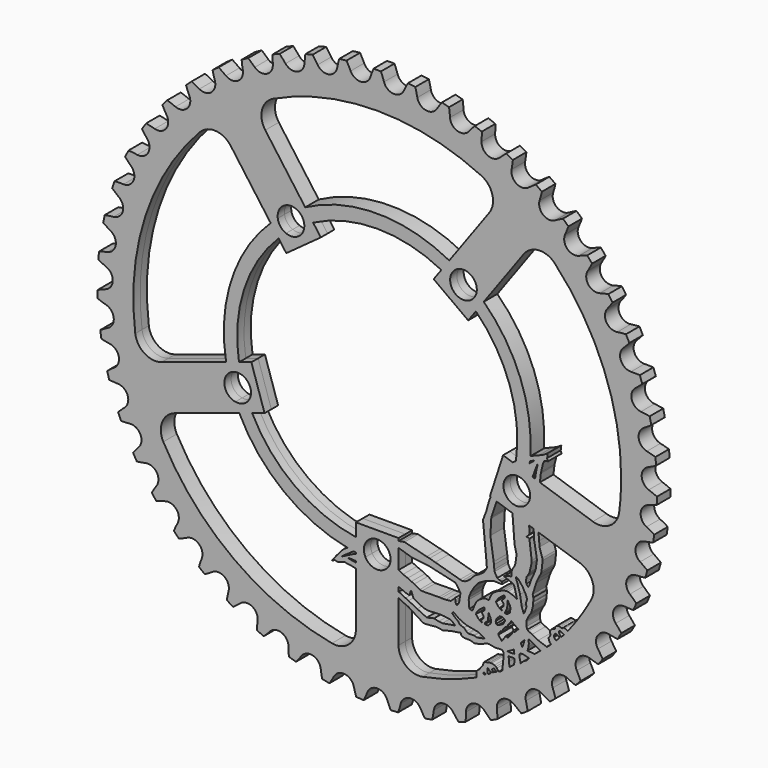
from build123d import *

# Parameters (mm, degrees)
F0_R     = 95.23914061
F2_DEPTH = 3.175
F3_DEPTH = 3.175


# Not quite as in the source:
# - a length typed as a fraction of an inch, garbled in the dataset ("3 / 203.2 mm" for 3/8 in), is restored


with BuildPart() as f2:
    # F0 (on Front) → F2 (new body, symmetric)
    with BuildSketch(Plane.XZ):
        with BuildLine():
            ThreePointArc((1.3974512393, 104.8471286678), (0, 104.8564411939), (-1.3974512393, 104.8471286678))
            ThreePointArc((-1.3974512393, 104.8471286678), (-1.9989055088, 103.3019703404), (-2.5462079028, 101.7368116953))
            ThreePointArc((-2.5462079028, 101.7368116953), (-3.9052398194, 99.8191421504), (-6.1056801538, 98.9930146972))
            ThreePointArc((-6.1056801538, 98.9930146972), (-8.3909636625, 99.5424721739), (-9.9753539423, 101.2785976519))
            ThreePointArc((-9.9753539423, 101.2785976519), (-10.7108477336, 102.7646361365), (-11.4976251519, 104.2241712642))
            ThreePointArc((-11.4976251519, 104.2241712642), (-12.8856288235, 104.061682812), (-14.2713436942, 103.880710476))
            ThreePointArc((-14.2713436942, 103.880710476), (-14.6783573813, 102.2733519742), (-15.0291718315, 100.6527993782))
            ThreePointArc((-15.0291718315, 100.6527993782), (-16.1422438465, 98.5826556819), (-18.224484574, 97.4923815023))
            ThreePointArc((-18.224484574, 97.4923815023), (-20.5599686886, 97.7568397874), (-22.34569959, 99.2851033058))
            ThreePointArc((-22.34569959, 99.2851033058), (-23.2582354424, 100.6694948013), (-24.2184092659, 102.0212816645))
            ThreePointArc((-24.2184092659, 102.0212816645), (-25.5759246489, 101.6894553933), (-26.9288971262, 101.3395666036))
            ThreePointArc((-26.9288971262, 101.3395666036), (-27.1353003181, 99.6943738437), (-27.2843088352, 98.0429932223))
            ThreePointArc((-27.2843088352, 98.0429932223), (-28.1345479113, 95.8517566428), (-30.0670243851, 94.5138631821))
            ThreePointArc((-30.0670243851, 94.5138631821), (-32.417305547, 94.4893133574), (-34.3773072098, 95.7865479992))
            ThreePointArc((-34.3773072098, 95.7865479992), (-35.45305201, 97.0483065417), (-36.5720669823, 98.2718534296))
            ThreePointArc((-36.5720669823, 98.2718534296), (-37.8785155273, 97.7757194874), (-39.1782359275, 97.2622182014))
            ThreePointArc((-39.1782359275, 97.2622182014), (-39.1808997623, 95.6041306286), (-39.125843529, 93.9469552287))
            ThreePointArc((-39.125843529, 93.9469552287), (-39.7003609085, 91.667842679), (-41.4537787551, 90.1026110382))
            ThreePointArc((-41.4537787551, 90.1026110382), (-43.7832290977, 89.7894252541), (-45.8877898946, 90.8359662645))
            ThreePointArc((-45.8877898946, 90.8359662645), (-47.110436448, 91.9559648806), (-48.3713294427, 93.0327240695))
            ThreePointArc((-48.3713294427, 93.0327240695), (-49.6069067216, 92.3798033412), (-50.8336726082, 91.7104737148))
            ThreePointArc((-50.8336726082, 91.7104737148), (-50.632556705, 90.0646262467), (-50.3742703176, 88.4267771581))
            ThreePointArc((-50.3742703176, 88.4267771581), (-50.6643569028, 86.0943376612), (-52.2121360949, 84.3254951565))
            ThreePointArc((-52.2121360949, 84.3254951565), (-54.4854435255, 83.7284209902), (-56.70266046, 84.5084038742))
            ThreePointArc((-56.70266046, 84.5084038742), (-58.0536746912, 85.4696645266), (-59.4373318558, 86.3833134448))
            ThreePointArc((-59.4373318558, 86.3833134448), (-60.5833077764, 85.5835035431), (-61.7185226292, 84.7684919313))
            ThreePointArc((-61.7185226292, 84.7684919313), (-61.3166757, 83.1598339377), (-60.8590745169, 81.5661392831))
            ThreePointArc((-60.8590745169, 81.5661392831), (-60.8603328907, 79.2157302442), (-62.1790106736, 77.2700907249))
            ThreePointArc((-62.1790106736, 77.2700907249), (-64.3617141688, 76.3981792122), (-66.6579764924, 76.8997802243))
            ThreePointArc((-66.6579764924, 76.8997802243), (-68.1168784028, 77.6877311814), (-69.6023249051, 78.4244198426))
            ThreePointArc((-69.6023249051, 78.4244198426), (-70.6413276406, 77.4898450703), (-71.6677827595, 76.5415062183))
            ThreePointArc((-71.6677827595, 76.5415062183), (-71.0712963941, 74.9944233147), (-70.4213171828, 73.4690418805))
            ThreePointArc((-70.4213171828, 73.4690418805), (-70.1337282697, 71.1362931047), (-71.2033148323, 69.0433504827))
            ThreePointArc((-71.2033148323, 69.0433504827), (-73.2623268321, 67.9098189133), (-75.6028255485, 68.1254342936))
            ThreePointArc((-75.6028255485, 68.1254342936), (-77.1474996722, 68.7281310219), (-78.7122176575, 69.276691977))
            ThreePointArc((-78.7122176575, 69.276691977), (-79.6284969855, 68.221519535), (-80.5306323574, 67.1542292932))
            ThreePointArc((-80.5306323574, 67.1542292932), (-79.748548681, 65.6921736793), (-78.9160444638, 64.2582286932))
            ThreePointArc((-78.9160444638, 64.2582286932), (-78.3439678185, 61.9785022741), (-79.1482493188, 59.7699834261))
            ThreePointArc((-79.1482493188, 59.7699834261), (-81.0523573, 58.3920149832), (-83.4016128346, 58.3183762222))
            ThreePointArc((-83.4016128346, 58.3183762222), (-85.0086434865, 58.7266824538), (-86.628913425, 59.0788000779))
            ThreePointArc((-86.628913425, 59.0788000779), (-87.408579485, 57.9190253048), (-88.172719657, 56.7489627052))
            ThreePointArc((-88.172719657, 56.7489627052), (-87.2168942611, 55.3940976539), (-86.2144849533, 54.0733262601))
            ThreePointArc((-86.2144849533, 54.0733262601), (-85.3665926745, 51.8811805265), (-85.8933770249, 49.5905643469))
            ThreePointArc((-85.8933770249, 49.5905643469), (-87.6137166516, 47.9890476274), (-89.9361166851, 47.6272710137))
            ThreePointArc((-89.9361166851, 47.6272710137), (-91.5811429185, 47.8349972424), (-93.2324031697, 47.9853337911))
            ThreePointArc((-93.2324031697, 47.9853337911), (-93.8636370189, 46.7385376903), (-94.478198405, 45.4834396894))
            ThreePointArc((-94.478198405, 45.4834396894), (-93.3631206282, 44.2563035737), (-92.2060017332, 43.0687273203))
            ThreePointArc((-92.2060017332, 43.0687273203), (-91.0951470036, 40.9973929669), (-91.3364486902, 38.6594028621))
            ThreePointArc((-91.3364486902, 38.6594028621), (-92.8469413671, 36.858615227), (-95.1072806824, 36.2141849253))
            ThreePointArc((-95.1072806824, 36.2141849253), (-96.7653655766, 36.2181822331), (-98.4225847182, 36.1644587577))
            ThreePointArc((-98.4225847182, 36.1644587577), (-98.8958174949, 34.8495414871), (-99.351483971, 33.5284340911))
            ThreePointArc((-99.351483971, 33.5284340911), (-98.0940572557, 32.4476290436), (-96.7997695163, 31.4112503761))
            ThreePointArc((-96.7997695163, 31.4112503761), (-95.4427917614, 29.4921267203), (-95.3949528966, 27.1422042371))
            ThreePointArc((-95.3949528966, 27.1422042371), (-96.6727010946, 25.1694437913), (-98.8367152516, 24.252128708))
            ThreePointArc((-98.8367152516, 24.252128708), (-100.4827239298, 24.0523364999), (-102.1207802088, 23.7953673935))
            ThreePointArc((-102.1207802088, 23.7953673935), (-102.4288381865, 22.4322617587), (-102.7187023133, 21.065171609))
            ThreePointArc((-102.7187023133, 21.065171609), (-101.3379879668, 20.1470815326), (-99.9261514659, 19.2776108951))
            ThreePointArc((-99.9261514659, 19.2776108951), (-98.343621085, 17.5397898952), (-98.0073668573, 15.2135574631))
            ThreePointArc((-98.0073668573, 15.2135574631), (-99.0330012161, 13.0987292441), (-101.0678859662, 11.9224349409))
            ThreePointArc((-101.0678859662, 11.9224349409), (-102.6768666145, 11.5218818629), (-104.2709287676, 11.0655625153))
            ThreePointArc((-104.2709287676, 11.0655625153), (-104.4091421014, 9.6749318081), (-104.5288098342, 8.2825825979))
            ThreePointArc((-104.5288098342, 8.2825825979), (-103.0457380786, 7.5411248023), (-101.5377548183, 6.8517424834))
            ThreePointArc((-101.5377548183, 6.8517424834), (-99.753661359, 5.3215677344), (-99.1340890397, 3.0542886658))
            ThreePointArc((-99.1340890397, 3.0542886658), (-99.8920619879, 0.8294513136), (-101.7669705525, -0.5879907869))
            ThreePointArc((-101.7669705525, -0.5879907869), (-103.3145326645, -1.1832327583), (-104.8404363343, -1.831985011))
            ThreePointArc((-104.8404363343, -1.831985011), (-104.8067098509, -3.2290602466), (-104.7543671488, -4.6255619225))
            ThreePointArc((-104.7543671488, -4.6255619225), (-103.1914198401, -5.1791476929), (-101.6101493096, -5.67799136))
            ThreePointArc((-101.6101493096, -5.67799136), (-99.6515378101, -6.9773239687), (-98.758039484, -9.1512800343))
            ThreePointArc((-98.758039484, -9.1512800343), (-99.2368609244, -11.4524002533), (-100.9233716008, -13.0895031738))
            ThreePointArc((-100.9233716008, -13.0895031738), (-102.3860557123, -13.870410777), (-103.8206697546, -14.701761512))
            ThreePointArc((-103.8206697546, -14.701761512), (-103.6155147131, -16.0841030394), (-103.3919550381, -17.4635876392))
            ThreePointArc((-103.3919550381, -17.4635876392), (-101.7728248644, -17.8209095885), (-100.142237513, -18.1216526423))
            ThreePointArc((-100.142237513, -18.1216526423), (-98.0387985272, -19.1704465528), (-96.8849187181, -21.2181246574))
            ThreePointArc((-96.8849187181, -21.2181246574), (-97.0773302057, -23.5606451062), (-98.5498772112, -25.3925920352))
            ThreePointArc((-98.5498772112, -25.3925920352), (-99.9055105221, -26.3473275071), (-101.2270876503, -27.3486742946))
            ThreePointArc((-101.2270876503, -27.3486742946), (-100.8536139921, -28.6953272254), (-100.4622262811, -30.0368831687))
            ThreePointArc((-100.4622262811, -30.0368831687), (-98.8114576053, -30.1925246603), (-97.1562714752, -30.2906081427))
            ThreePointArc((-97.1562714752, -30.2906081427), (-94.9398909938, -31.0729647084), (-93.5431213435, -32.9633241392))
            ThreePointArc((-93.5431213435, -32.9633241392), (-93.4462061162, -35.3117345958), (-94.6824671393, -37.3107550852))
            ThreePointArc((-94.6824671393, -37.3107550852), (-95.9104996304, -38.4248456091), (-97.0990060825, -39.5810090527))
            ThreePointArc((-97.0990060825, -39.5810090527), (-96.5628752875, -40.8715595011), (-96.0095925791, -42.1548501673))
            ThreePointArc((-96.0095925791, -42.1548501673), (-94.3522093717, -42.1064518349), (-92.6975153974, -42.0003889001))
            ThreePointArc((-92.6975153974, -42.0003889001), (-90.4017914894, -42.504448393), (-88.7833056019, -44.2088332281))
            ThreePointArc((-88.7833056019, -44.2088332281), (-88.3985327959, -46.5275341837), (-89.3797673795, -48.6633251205))
            ThreePointArc((-89.3797673795, -48.6633251205), (-90.4615833302, -49.9198822198), (-91.4990025598, -51.2133360601))
            ThreePointArc((-91.4990025598, -51.2133360601), (-90.8083418243, -52.4282205969), (-90.1015513205, -53.6337926077))
            ThreePointArc((-90.1015513205, -53.6337926077), (-88.4626778214, -53.3820881206), (-86.8335594768, -53.0734865747))
            ThreePointArc((-86.8335594768, -53.0734865747), (-84.4932929765, -53.2916079667), (-82.6776254481, -54.7841814692))
            ThreePointArc((-82.6776254481, -54.7841814692), (-82.0108278269, -57.0380237809), (-82.722161455, -59.2782087517))
            ThreePointArc((-82.722161455, -59.2782087517), (-83.6413616381, -60.6581843016), (-84.5119674272, -62.0693210969))
            ThreePointArc((-84.5119674272, -62.0693210969), (-83.677246464, -63.1901233109), (-82.8276623883, -64.2997014234))
            ThreePointArc((-82.8276623883, -64.2997014234), (-81.2321422492, -63.8485063651), (-79.6532953078, -63.342044293))
            ThreePointArc((-79.6532953078, -63.342044293), (-77.3039622698, -63.270921086), (-75.3186367695, -64.5290573631))
            ThreePointArc((-75.3186367695, -64.5290573631), (-74.3799223052, -66.683875079), (-74.8105718852, -68.9944951631))
            ThreePointArc((-74.8105718852, -68.9944951631), (-75.5532221629, -70.476970141), (-76.2438170152, -71.9843984958))
            ThreePointArc((-76.2438170152, -71.9843984958), (-75.2776893432, -72.9941281679), (-74.2981905242, -73.990892309))
            ThreePointArc((-74.2981905242, -73.990892309), (-72.770210204, -73.3470463367), (-71.265568376, -72.6504011871))
            ThreePointArc((-71.265568376, -72.6504011871), (-68.9427822944, -72.2911115366), (-66.817894333, -73.2957385248))
            ThreePointArc((-66.817894333, -73.2957385248), (-65.6214929802, -75.3188668047), (-65.7649303033, -77.664895357))
            ThreePointArc((-65.7649303033, -77.664895357), (-66.3197728544, -79.2273969532), (-66.8198880558, -80.8082657904))
            ThreePointArc((-66.8198880558, -80.8082657904), (-65.7369991858, -81.691616448), (-64.6424338271, -82.5604566893))
            ThreePointArc((-64.6424338271, -82.5604566893), (-63.20515595, -81.7337198516), (-61.7975280718, -80.857452055))
            ThreePointArc((-61.7975280718, -80.857452055), (-59.5365000158, -80.2154424257), (-57.3042607288, -80.9513310039))
            ThreePointArc((-57.3042607288, -80.9513310039), (-55.8683087124, -82.8121012854), (-55.7223594151, -85.1579749044))
            ThreePointArc((-55.7223594151, -85.1579749044), (-56.0809833921, -86.7768171877), (-56.3830377061, -88.407162147))
            ThreePointArc((-56.3830377061, -88.407162147), (-55.1998031293, -89.1507430946), (-54.006763726, -89.8784887038))
            ThreePointArc((-54.006763726, -89.8784887038), (-52.6819759595, -88.8813934884), (-51.3927002349, -87.8387863712))
            ThreePointArc((-51.3927002349, -87.8387863712), (-49.2277050852, -86.9237889748), (-46.9219529448, -87.3797838223))
            ThreePointArc((-46.9219529448, -87.3797838223), (-45.2682178335, -89.0499887246), (-44.8350943583, -91.3601463576))
            ThreePointArc((-44.8350943583, -91.3601463576), (-44.9920633874, -93.0107893289), (-45.0914779783, -94.6658960427))
            ThreePointArc((-45.0914779783, -94.6658960427), (-43.825834325, -95.2584353512), (-42.5524061384, -95.8340544466))
            ThreePointArc((-42.5524061384, -95.8340544466), (-41.3601909146, -94.6817158006), (-40.2088114494, -93.488574224))
            ThreePointArc((-40.2088114494, -93.488574224), (-38.1726683254, -92.3144594882), (-35.8283561837, -92.483648188))
            ThreePointArc((-35.8283561837, -92.483648188), (-33.9819069162, -93.9379691074), (-33.2681749735, -96.1773911194))
            ThreePointArc((-33.2681749735, -96.1773911194), (-33.2211095641, -97.834812714), (-33.1163774082, -99.4895914516))
            ThreePointArc((-33.1163774082, -99.4895914516), (-31.7875105459, -99.9221068289), (-30.4529974492, -100.3368736118))
            ThreePointArc((-30.4529974492, -100.3368736118), (-29.4114275356, -99.0467598146), (-28.4153980688, -97.7211705886))
            ThreePointArc((-28.4153980688, -97.7211705886), (-26.5389728249, -96.305736896), (-24.1916380643, -96.1855547198))
            ThreePointArc((-24.1916380643, -96.1855547198), (-22.1804649293, -97.4019456336), (-21.1969439678, -99.5366846697))
            ThreePointArc((-21.1969439678, -99.5366846697), (-20.9465575835, -101.1757600656), (-20.6392663135, -102.8051260681))
            ThreePointArc((-20.6392663135, -102.8051260681), (-19.2673205093, -103.0710610221), (-17.8919523608, -103.3186880509))
            ThreePointArc((-17.8919523608, -103.3186880509), (-17.0168168956, -101.9103559124), (-16.1912362186, -100.4724136185))
            ThreePointArc((-16.1912362186, -100.4724136185), (-14.5029735487, -98.8371175011), (-12.1881993714, -98.4293862882))
            ThreePointArc((-12.1881993714, -98.4293862882), (-10.0427897036, -99.38940795), (-8.8043888985, -101.3871035425))
            ThreePointArc((-8.8043888985, -101.3871035425), (-8.3544771417, -102.9829860275), (-7.84928498, -104.5622397672))
            ThreePointArc((-7.84928498, -104.5622397672), (-6.4550575339, -104.6575629951), (-5.0596835126, -104.7342964964))
            ThreePointArc((-5.0596835126, -104.7342964964), (-4.3642486574, -103.2290948963), (-3.7216317317, -101.7005972739))
            ThreePointArc((-3.7216317317, -101.7005972739), (-2.247123977, -99.8702281539), (0, -99.1811286939))
            ThreePointArc((0, -99.1811286939), (2.247123977, -99.8702281539), (3.7216317317, -101.7005972739))
            ThreePointArc((3.7216317317, -101.7005972739), (4.3642486574, -103.2290948963), (5.0596835126, -104.7342964964))
            ThreePointArc((5.0596835126, -104.7342964964), (6.4550575339, -104.6575629951), (7.84928498, -104.5622397672))
            ThreePointArc((7.84928498, -104.5622397672), (8.3544771417, -102.9829860275), (8.8043888985, -101.3871035425))
            ThreePointArc((8.8043888985, -101.3871035425), (10.0427897036, -99.38940795), (12.1881993714, -98.4293862882))
            ThreePointArc((12.1881993714, -98.4293862882), (14.5029735487, -98.8371175011), (16.1912362186, -100.4724136185))
            ThreePointArc((16.1912362186, -100.4724136185), (17.0168168956, -101.9103559124), (17.8919523608, -103.3186880509))
            ThreePointArc((17.8919523608, -103.3186880509), (19.2673205093, -103.0710610221), (20.6392663135, -102.8051260681))
            ThreePointArc((20.6392663135, -102.8051260681), (20.9465575835, -101.1757600656), (21.1969439678, -99.5366846697))
            ThreePointArc((21.1969439678, -99.5366846697), (22.1804649293, -97.4019456336), (24.1916380643, -96.1855547198))
            ThreePointArc((24.1916380643, -96.1855547198), (26.5389728249, -96.305736896), (28.4153980688, -97.7211705886))
            ThreePointArc((28.4153980688, -97.7211705886), (29.4114275356, -99.0467598146), (30.4529974492, -100.3368736118))
            ThreePointArc((30.4529974492, -100.3368736118), (31.7875105459, -99.9221068289), (33.1163774082, -99.4895914516))
            ThreePointArc((33.1163774082, -99.4895914516), (33.2211095641, -97.834812714), (33.2681749735, -96.1773911194))
            ThreePointArc((33.2681749735, -96.1773911194), (33.9819069162, -93.9379691074), (35.8283561837, -92.483648188))
            ThreePointArc((35.8283561837, -92.483648188), (38.1726683254, -92.3144594882), (40.2088114494, -93.488574224))
            ThreePointArc((40.2088114494, -93.488574224), (41.3601909146, -94.6817158006), (42.5524061384, -95.8340544466))
            ThreePointArc((42.5524061384, -95.8340544466), (43.825834325, -95.2584353512), (45.0914779783, -94.6658960427))
            ThreePointArc((45.0914779783, -94.6658960427), (44.9920633874, -93.0107893289), (44.8350943583, -91.3601463576))
            ThreePointArc((44.8350943583, -91.3601463576), (45.2682178335, -89.0499887246), (46.9219529448, -87.3797838223))
            ThreePointArc((46.9219529448, -87.3797838223), (49.2277050852, -86.9237889748), (51.3927002349, -87.8387863712))
            ThreePointArc((51.3927002349, -87.8387863712), (52.6819759595, -88.8813934884), (54.006763726, -89.8784887038))
            ThreePointArc((54.006763726, -89.8784887038), (55.1998031293, -89.1507430946), (56.3830377061, -88.407162147))
            ThreePointArc((56.3830377061, -88.407162147), (56.0809833921, -86.7768171877), (55.7223594151, -85.1579749044))
            ThreePointArc((55.7223594151, -85.1579749044), (55.8683087124, -82.8121012854), (57.3042607288, -80.9513310039))
            ThreePointArc((57.3042607288, -80.9513310039), (59.5365000158, -80.2154424257), (61.7975280718, -80.857452055))
            ThreePointArc((61.7975280718, -80.857452055), (63.20515595, -81.7337198516), (64.6424338271, -82.5604566893))
            ThreePointArc((64.6424338271, -82.5604566893), (65.7369991858, -81.691616448), (66.8198880558, -80.8082657904))
            ThreePointArc((66.8198880558, -80.8082657904), (66.3197728544, -79.2273969532), (65.7649303033, -77.664895357))
            ThreePointArc((65.7649303033, -77.664895357), (65.6214929802, -75.3188668047), (66.817894333, -73.2957385248))
            ThreePointArc((66.817894333, -73.2957385248), (68.9427822944, -72.2911115366), (71.265568376, -72.6504011871))
            ThreePointArc((71.265568376, -72.6504011871), (72.770210204, -73.3470463367), (74.2981905242, -73.990892309))
            ThreePointArc((74.2981905242, -73.990892309), (75.2776893432, -72.9941281679), (76.2438170152, -71.9843984958))
            ThreePointArc((76.2438170152, -71.9843984958), (75.5532221629, -70.476970141), (74.8105718852, -68.9944951631))
            ThreePointArc((74.8105718852, -68.9944951631), (74.3799223052, -66.683875079), (75.3186367695, -64.5290573631))
            ThreePointArc((75.3186367695, -64.5290573631), (77.3039622698, -63.270921086), (79.6532953078, -63.342044293))
            ThreePointArc((79.6532953078, -63.342044293), (81.2321422492, -63.8485063651), (82.8276623883, -64.2997014234))
            ThreePointArc((82.8276623883, -64.2997014234), (83.677246464, -63.1901233109), (84.5119674272, -62.0693210969))
            ThreePointArc((84.5119674272, -62.0693210969), (83.6413616381, -60.6581843016), (82.722161455, -59.2782087517))
            ThreePointArc((82.722161455, -59.2782087517), (82.0108278269, -57.0380237809), (82.6776254481, -54.7841814692))
            ThreePointArc((82.6776254481, -54.7841814692), (84.4932929765, -53.2916079667), (86.8335594768, -53.0734865747))
            ThreePointArc((86.8335594768, -53.0734865747), (88.4626778214, -53.3820881206), (90.1015513205, -53.6337926077))
            ThreePointArc((90.1015513205, -53.6337926077), (90.8083418243, -52.4282205969), (91.4990025598, -51.2133360601))
            ThreePointArc((91.4990025598, -51.2133360601), (90.4615833302, -49.9198822198), (89.3797673795, -48.6633251205))
            ThreePointArc((89.3797673795, -48.6633251205), (88.3985327959, -46.5275341837), (88.7833056019, -44.2088332281))
            ThreePointArc((88.7833056019, -44.2088332281), (90.4017914894, -42.504448393), (92.6975153974, -42.0003889001))
            ThreePointArc((92.6975153974, -42.0003889001), (94.3522093717, -42.1064518349), (96.0095925791, -42.1548501673))
            ThreePointArc((96.0095925791, -42.1548501673), (96.5628752875, -40.8715595011), (97.0990060825, -39.5810090527))
            ThreePointArc((97.0990060825, -39.5810090527), (95.9104996304, -38.4248456091), (94.6824671393, -37.3107550852))
            ThreePointArc((94.6824671393, -37.3107550852), (93.4462061162, -35.3117345958), (93.5431213435, -32.9633241392))
            ThreePointArc((93.5431213435, -32.9633241392), (94.9398909938, -31.0729647084), (97.1562714752, -30.2906081427))
            ThreePointArc((97.1562714752, -30.2906081427), (98.8114576053, -30.1925246603), (100.4622262811, -30.0368831687))
            ThreePointArc((100.4622262811, -30.0368831687), (100.8536139921, -28.6953272254), (101.2270876503, -27.3486742946))
            ThreePointArc((101.2270876503, -27.3486742946), (99.9055105221, -26.3473275071), (98.5498772112, -25.3925920352))
            ThreePointArc((98.5498772112, -25.3925920352), (97.0773302057, -23.5606451062), (96.8849187181, -21.2181246574))
            ThreePointArc((96.8849187181, -21.2181246574), (98.0387985272, -19.1704465528), (100.142237513, -18.1216526423))
            ThreePointArc((100.142237513, -18.1216526423), (101.7728248644, -17.8209095885), (103.3919550381, -17.4635876392))
            ThreePointArc((103.3919550381, -17.4635876392), (103.6155147131, -16.0841030394), (103.8206697546, -14.701761512))
            ThreePointArc((103.8206697546, -14.701761512), (102.3860557123, -13.870410777), (100.9233716008, -13.0895031738))
            ThreePointArc((100.9233716008, -13.0895031738), (99.2368609244, -11.4524002533), (98.758039484, -9.1512800343))
            ThreePointArc((98.758039484, -9.1512800343), (99.6515378101, -6.9773239687), (101.6101493096, -5.67799136))
            ThreePointArc((101.6101493096, -5.67799136), (103.1914198401, -5.1791476929), (104.7543671488, -4.6255619225))
            ThreePointArc((104.7543671488, -4.6255619225), (104.8067098509, -3.2290602466), (104.8404363343, -1.831985011))
            ThreePointArc((104.8404363343, -1.831985011), (103.3145326645, -1.1832327583), (101.7669705525, -0.5879907869))
            ThreePointArc((101.7669705525, -0.5879907869), (99.8920619879, 0.8294513136), (99.1340890397, 3.0542886658))
            ThreePointArc((99.1340890397, 3.0542886658), (99.753661359, 5.3215677344), (101.5377548183, 6.8517424834))
            ThreePointArc((101.5377548183, 6.8517424834), (103.0457380786, 7.5411248023), (104.5288098342, 8.2825825979))
            ThreePointArc((104.5288098342, 8.2825825979), (104.4091421014, 9.6749318081), (104.2709287676, 11.0655625153))
            ThreePointArc((104.2709287676, 11.0655625153), (102.6768666145, 11.5218818629), (101.0678859662, 11.9224349409))
            ThreePointArc((101.0678859662, 11.9224349409), (99.0330012161, 13.0987292441), (98.0073668573, 15.2135574631))
            ThreePointArc((98.0073668573, 15.2135574631), (98.343621085, 17.5397898952), (99.9261514659, 19.2776108951))
            ThreePointArc((99.9261514659, 19.2776108951), (101.3379879668, 20.1470815326), (102.7187023133, 21.065171609))
            ThreePointArc((102.7187023133, 21.065171609), (102.4288381865, 22.4322617587), (102.1207802088, 23.7953673935))
            ThreePointArc((102.1207802088, 23.7953673935), (100.4827239298, 24.0523364999), (98.8367152516, 24.252128708))
            ThreePointArc((98.8367152516, 24.252128708), (96.6727010946, 25.1694437913), (95.3949528966, 27.1422042371))
            ThreePointArc((95.3949528966, 27.1422042371), (95.4427917614, 29.4921267203), (96.7997695163, 31.4112503761))
            ThreePointArc((96.7997695163, 31.4112503761), (98.0940572557, 32.4476290436), (99.351483971, 33.5284340911))
            ThreePointArc((99.351483971, 33.5284340911), (98.8958174949, 34.8495414871), (98.4225847182, 36.1644587577))
            ThreePointArc((98.4225847182, 36.1644587577), (96.7653655766, 36.2181822331), (95.1072806824, 36.2141849253))
            ThreePointArc((95.1072806824, 36.2141849253), (92.8469413671, 36.858615227), (91.3364486902, 38.6594028621))
            ThreePointArc((91.3364486902, 38.6594028621), (91.0951470036, 40.9973929669), (92.2060017332, 43.0687273203))
            ThreePointArc((92.2060017332, 43.0687273203), (93.3631206282, 44.2563035737), (94.478198405, 45.4834396894))
            ThreePointArc((94.478198405, 45.4834396894), (93.8636370189, 46.7385376903), (93.2324031697, 47.9853337911))
            ThreePointArc((93.2324031697, 47.9853337911), (91.5811429185, 47.8349972424), (89.9361166851, 47.6272710137))
            ThreePointArc((89.9361166851, 47.6272710137), (87.6137166516, 47.9890476274), (85.8933770249, 49.5905643469))
            ThreePointArc((85.8933770249, 49.5905643469), (85.3665926745, 51.8811805265), (86.2144849533, 54.0733262601))
            ThreePointArc((86.2144849533, 54.0733262601), (87.2168942611, 55.3940976539), (88.172719657, 56.7489627052))
            ThreePointArc((88.172719657, 56.7489627052), (87.408579485, 57.9190253048), (86.628913425, 59.0788000779))
            ThreePointArc((86.628913425, 59.0788000779), (85.0086434865, 58.7266824538), (83.4016128346, 58.3183762222))
            ThreePointArc((83.4016128346, 58.3183762222), (81.0523573, 58.3920149832), (79.1482493188, 59.7699834261))
            ThreePointArc((79.1482493188, 59.7699834261), (78.3439678185, 61.9785022741), (78.9160444638, 64.2582286932))
            ThreePointArc((78.9160444638, 64.2582286932), (79.748548681, 65.6921736793), (80.5306323574, 67.1542292932))
            ThreePointArc((80.5306323574, 67.1542292932), (79.6284969855, 68.221519535), (78.7122176575, 69.276691977))
            ThreePointArc((78.7122176575, 69.276691977), (77.1474996722, 68.7281310219), (75.6028255485, 68.1254342936))
            ThreePointArc((75.6028255485, 68.1254342936), (73.2623268321, 67.9098189133), (71.2033148323, 69.0433504827))
            ThreePointArc((71.2033148323, 69.0433504827), (70.1337282697, 71.1362931047), (70.4213171828, 73.4690418805))
            ThreePointArc((70.4213171828, 73.4690418805), (71.0712963941, 74.9944233147), (71.6677827595, 76.5415062183))
            ThreePointArc((71.6677827595, 76.5415062183), (70.6413276406, 77.4898450703), (69.6023249051, 78.4244198426))
            ThreePointArc((69.6023249051, 78.4244198426), (68.1168784028, 77.6877311814), (66.6579764924, 76.8997802243))
            ThreePointArc((66.6579764924, 76.8997802243), (64.3617141688, 76.3981792122), (62.1790106736, 77.2700907249))
            ThreePointArc((62.1790106736, 77.2700907249), (60.8603328907, 79.2157302442), (60.8590745169, 81.5661392831))
            ThreePointArc((60.8590745169, 81.5661392831), (61.3166757, 83.1598339377), (61.7185226292, 84.7684919313))
            ThreePointArc((61.7185226292, 84.7684919313), (60.5833077764, 85.5835035431), (59.4373318558, 86.3833134448))
            ThreePointArc((59.4373318558, 86.3833134448), (58.0536746912, 85.4696645266), (56.70266046, 84.5084038742))
            ThreePointArc((56.70266046, 84.5084038742), (54.4854435255, 83.7284209902), (52.2121360949, 84.3254951565))
            ThreePointArc((52.2121360949, 84.3254951565), (50.6643569028, 86.0943376612), (50.3742703176, 88.4267771581))
            ThreePointArc((50.3742703176, 88.4267771581), (50.632556705, 90.0646262467), (50.8336726082, 91.7104737148))
            ThreePointArc((50.8336726082, 91.7104737148), (49.6069067216, 92.3798033412), (48.3713294427, 93.0327240695))
            ThreePointArc((48.3713294427, 93.0327240695), (47.110436448, 91.9559648806), (45.8877898946, 90.8359662645))
            ThreePointArc((45.8877898946, 90.8359662645), (43.7832290977, 89.7894252541), (41.4537787551, 90.1026110382))
            ThreePointArc((41.4537787551, 90.1026110382), (39.7003609085, 91.667842679), (39.125843529, 93.9469552287))
            ThreePointArc((39.125843529, 93.9469552287), (39.1808997623, 95.6041306286), (39.1782359275, 97.2622182014))
            ThreePointArc((39.1782359275, 97.2622182014), (37.8785155273, 97.7757194874), (36.5720669823, 98.2718534296))
            ThreePointArc((36.5720669823, 98.2718534296), (35.45305201, 97.0483065417), (34.3773072098, 95.7865479992))
            ThreePointArc((34.3773072098, 95.7865479992), (32.417305547, 94.4893133574), (30.0670243851, 94.5138631821))
            ThreePointArc((30.0670243851, 94.5138631821), (28.1345479113, 95.8517566428), (27.2843088352, 98.0429932223))
            ThreePointArc((27.2843088352, 98.0429932223), (27.1353003181, 99.6943738437), (26.9288971262, 101.3395666036))
            ThreePointArc((26.9288971262, 101.3395666036), (25.5759246489, 101.6894553933), (24.2184092659, 102.0212816645))
            ThreePointArc((24.2184092659, 102.0212816645), (23.2582354424, 100.6694948013), (22.34569959, 99.2851033058))
            ThreePointArc((22.34569959, 99.2851033058), (20.5599686886, 97.7568397874), (18.224484574, 97.4923815023))
            ThreePointArc((18.224484574, 97.4923815023), (16.1422438465, 98.5826556819), (15.0291718315, 100.6527993782))
            ThreePointArc((15.0291718315, 100.6527993782), (14.6783573813, 102.2733519742), (14.2713436942, 103.880710476))
            ThreePointArc((14.2713436942, 103.880710476), (12.8856288235, 104.061682812), (11.4976251519, 104.2241712642))
            ThreePointArc((11.4976251519, 104.2241712642), (10.7108477336, 102.7646361365), (9.9753539423, 101.2785976519))
            ThreePointArc((9.9753539423, 101.2785976519), (8.3909636625, 99.5424721739), (6.1056801538, 98.9930146972))
            ThreePointArc((6.1056801538, 98.9930146972), (3.9052398194, 99.8191421504), (2.5462079028, 101.7368116953))
            ThreePointArc((2.5462079028, 101.7368116953), (1.9989055088, 103.3019703404), (1.3974512393, 104.8471286678))
        make_face()
        Circle(F0_R, mode=Mode.SUBTRACT)
        Circle(F0_R)
        with BuildLine():
            ThreePointArc((16.99286117, -89.8361309382), (0, -91.42914061), (-16.99286117, -89.8361309382))
            ThreePointArc((-16.99286117, -89.8361309382), (-53.7407004803, -73.9677285346), (-80.1881548429, -43.922062515))
            ThreePointArc((-80.1881548429, -43.922062515), (-86.9542799564, -28.2531582296), (-90.6903206121, -11.5997198226))
            ThreePointArc((-90.6903206121, -11.5997198226), (-86.9542799564, 28.2531582296), (-66.551866358, 62.6908034479))
            ThreePointArc((-66.551866358, 62.6908034479), (-53.7407004803, 73.9677285346), (-39.0568394189, 82.6671098278))
            ThreePointArc((-39.0568394189, 82.6671098278), (0, 91.42914061), (39.0568394189, 82.6671098278))
            ThreePointArc((39.0568394189, 82.6671098278), (53.7407004803, 73.9677285346), (66.551866358, 62.6908034479))
            ThreePointArc((66.551866358, 62.6908034479), (84.9825502671, 33.7231953229), (91.42914061, 0))
            ThreePointArc((91.42914061, 0), (91.2442486623, -5.8116124043), (90.6903206121, -11.5997198226))
            ThreePointArc((90.6903206121, -11.5997198226), (86.9542799564, -28.2531582296), (80.1881548429, -43.922062515))
            ThreePointArc((80.1881548429, -43.922062515), (53.7407004803, -73.9677285346), (16.99286117, -89.8361309382))
        make_face(mode=Mode.SUBTRACT)
        with BuildLine():
            ThreePointArc((75.8805031971, -33.0667678427), (80.5858170493, -37.4819210974), (80.1881548429, -43.922062515))
            ThreePointArc((80.1881548429, -43.922062515), (86.9542799564, -28.2531582296), (90.6903206121, -11.5997198226))
            ThreePointArc((90.6903206121, -11.5997198226), (87.2266159471, -17.0436436559), (80.8247751071, -17.849863582))
            Line((80.8247751071, -17.849863582), (56.6260155483, -9.9872099769))
            ThreePointArc((56.6260155483, -9.9872099769), (56.2859359025, -11.7534428821), (55.8907793241, -13.5081748045))
            ThreePointArc((55.8907793241, -13.5081748045), (56.9402436835, -15.1135631331), (57.3081083962, -16.9959346906))
            ThreePointArc((57.3081083962, -16.9959346906), (49.2395161146, -20.9435594713), (51.0746118327, -12.1504743175))
            ThreePointArc((51.0746118327, -12.1504743175), (51.4807614826, -10.2947169547), (51.8195067214, -8.4254805889))
            Line((51.8195067214, -8.4254805889), (47.1717922209, -6.9153466053))
            Line((47.1717922209, -6.9153466053), (42.2275203109, -22.132250866))
            Line((42.2275203109, -22.132250866), (75.8805031971, -33.0667678427))
        make_face()
        with BuildLine():
            ThreePointArc((-4.2271352617, -52.3295454545), (1.3900222465, -50.1971010677), (5, -55))
            ThreePointArc((5, -55), (1.1998302287, -59.8539064085), (-4.4241629689, -57.3295454545))
            ThreePointArc((-4.4241629689, -57.3295454545), (-6.2151222962, -57.1631197088), (-8, -56.9407586883))
            Line((-8, -56.9407586883), (-8, -82.3848402378))
            ThreePointArc((-8, -82.3848402378), (-10.7450383291, -88.2242170266), (-16.99286117, -89.8361309382))
            ThreePointArc((-16.99286117, -89.8361309382), (0, -91.42914061), (16.99286117, -89.8361309382))
            ThreePointArc((16.99286117, -89.8361309382), (10.7450383291, -88.2242170266), (8, -82.3848402378))
            Line((8, -82.3848402378), (8, -47))
            Line((8, -47), (-8, -47))
            Line((-8, -47), (-8, -51.8868962263))
            ThreePointArc((-8, -51.8868962263), (-6.1175725383, -52.1423561631), (-4.2271352617, -52.3295454545))
        make_face()
        with BuildLine():
            ThreePointArc((-39.0568394189, 82.6671098278), (-53.7407004803, 73.9677285346), (-66.551866358, 62.6908034479))
            ThreePointArc((-66.551866358, 62.6908034479), (-60.5498122767, 65.0591158248), (-54.8967300593, 61.9484538129))
            Line((-54.8967300593, 61.9484538129), (-39.9410741663, 41.3637594331))
            ThreePointArc((-39.9410741663, 41.3637594331), (-38.6277782996, 42.592778069), (-37.2766843665, 43.7801188057))
            ThreePointArc((-37.2766843665, 43.7801188057), (-35.2671151375, 48.5410196625), (-30.1182383111, 48.9810342994))
            ThreePointArc((-30.1182383111, 48.9810342994), (-28.5714991801, 49.8990925228), (-26.9968022563, 50.7683234698))
            Line((-26.9968022563, 50.7683234698), (-41.9524581493, 71.3530178496))
            ThreePointArc((-41.9524581493, 71.3530178496), (-43.1639750498, 77.6906659551), (-39.0568394189, 82.6671098278))
        make_face()
        with BuildLine():
            ThreePointArc((66.551866358, 62.6908034479), (53.7407004803, 73.9677285346), (39.0568394189, 82.6671098278))
            ThreePointArc((39.0568394189, 82.6671098278), (43.1639750498, 77.6906659551), (41.9524581493, 71.3530178496))
            Line((41.9524581493, 71.3530178496), (26.9968022563, 50.7683234698))
            ThreePointArc((26.9968022563, 50.7683234698), (28.5714991801, 49.8990925228), (30.1182383111, 48.9810342994))
            ThreePointArc((30.1182383111, 48.9810342994), (34.9692348029, 48.7415060788), (37.3281888761, 44.4959346906))
            ThreePointArc((37.3281888761, 44.4959346906), (37.3152961264, 44.1371014788), (37.2766843665, 43.7801188057))
            ThreePointArc((37.2766843665, 43.7801188057), (38.6277782996, 42.592778069), (39.9410741663, 41.3637594331))
            Line((39.9410741663, 41.3637594331), (54.8967300593, 61.9484538129))
            ThreePointArc((54.8967300593, 61.9484538129), (60.5498122767, 65.0591158248), (66.551866358, 62.6908034479))
        make_face()
        with BuildLine():
            Line((-75.8805031971, -33.0667678427), (-51.6817436383, -25.2041142377))
            ThreePointArc((-51.6817436383, -25.2041142377), (-52.4447790792, -23.5753080009), (-53.1564962375, -21.923432846))
            ThreePointArc((-53.1564962375, -21.923432846), (-57.0633909777, -18.5410196625), (-55.8907793241, -13.5081748045))
            ThreePointArc((-55.8907793241, -13.5081748045), (-56.2859359025, -11.7534428821), (-56.6260155483, -9.9872099769))
            Line((-56.6260155483, -9.9872099769), (-80.8247751071, -17.849863582))
            ThreePointArc((-80.8247751071, -17.849863582), (-87.2266159471, -17.0436436559), (-90.6903206121, -11.5997198226))
            ThreePointArc((-90.6903206121, -11.5997198226), (-86.9542799564, -28.2531582296), (-80.1881548429, -43.922062515))
            ThreePointArc((-80.1881548429, -43.922062515), (-80.5858170493, -37.4819210974), (-75.8805031971, -33.0667678427))
        make_face()
        with BuildLine():
            Line((-8, -56.9407586883), (-8, -51.8868962263))
            ThreePointArc((-8, -51.8868962263), (-30.8587257454, -42.4733922047), (-46.8752348114, -23.6423848497))
            Line((-46.8752348114, -23.6423848497), (-51.6817436383, -25.2041142377))
            ThreePointArc((-51.6817436383, -25.2041142377), (-33.7976520068, -46.5184771766), (-8, -56.9407586883))
        make_face()
        with BuildLine():
            Line((-56.6260155483, -9.9872099769), (-51.8195067214, -8.4254805889))
            ThreePointArc((-51.8195067214, -8.4254805889), (-49.9304671055, 16.2233922047), (-36.9704883441, 37.2750988141))
            Line((-36.9704883441, 37.2750988141), (-39.9410741663, 41.3637594331))
            ThreePointArc((-39.9410741663, 41.3637594331), (-54.685749687, 17.7684771766), (-56.6260155483, -9.9872099769))
        make_face()
        with BuildLine():
            Line((-26.9968022563, 50.7683234698), (-24.0262164341, 46.6796628508))
            ThreePointArc((-24.0262164341, 46.6796628508), (0, 52.5), (24.0262164341, 46.6796628508))
            Line((24.0262164341, 46.6796628508), (26.9968022563, 50.7683234698))
            ThreePointArc((26.9968022563, 50.7683234698), (0, 57.5), (-26.9968022563, 50.7683234698))
        make_face()
        with BuildLine():
            Line((51.8195067214, -8.4254805889), (56.6260155483, -9.9872099769))
            ThreePointArc((56.6260155483, -9.9872099769), (54.685749687, 17.7684771766), (39.9410741663, 41.3637594331))
            Line((39.9410741663, 41.3637594331), (36.9704883441, 37.2750988141))
            ThreePointArc((36.9704883441, 37.2750988141), (49.9304671055, 16.2233922047), (51.8195067214, -8.4254805889))
        make_face()
        with BuildLine():
            ThreePointArc((27.3387108131, 44.8201393469), (25.6992878246, 45.7798711806), (24.0262164341, 46.6796628508))
            Line((24.0262164341, 46.6796628508), (21.1537709027, 42.726080754))
            Line((21.1537709027, 42.726080754), (34.0980428127, 33.3215167173))
            Line((34.0980428127, 33.3215167173), (36.9704883441, 37.2750988141))
            ThreePointArc((36.9704883441, 37.2750988141), (35.5977281203, 38.5882333448), (34.1783593416, 39.8508438144))
            ThreePointArc((34.1783593416, 39.8508438144), (29.3892626146, 40.4508497187), (27.3387108131, 44.8201393469))
        make_face()
        with BuildLine():
            ThreePointArc((-34.1783593416, 39.8508438144), (-35.5977281203, 38.5882333448), (-36.9704883441, 37.2750988141))
            Line((-36.9704883441, 37.2750988141), (-34.0980428127, 33.3215167173))
            Line((-34.0980428127, 33.3215167173), (-21.1537709027, 42.726080754))
            Line((-21.1537709027, 42.726080754), (-24.0262164341, 46.6796628508))
            ThreePointArc((-24.0262164341, 46.6796628508), (-25.6992878246, 45.7798711806), (-27.3387108131, 44.8201393469))
            ThreePointArc((-27.3387108131, 44.8201393469), (-27.3308200527, 44.6581223677), (-27.3281888761, 44.4959346906))
            ThreePointArc((-27.3281888761, 44.4959346906), (-29.5220217684, 40.3576468606), (-34.1783593416, 39.8508438144))
        make_face()
        with BuildLine():
            ThreePointArc((-48.4620985659, -20.1909633893), (-47.6998937252, -21.9310314076), (-46.8752348114, -23.6423848497))
            Line((-46.8752348114, -23.6423848497), (-42.2275203109, -22.132250866))
            Line((-42.2275203109, -22.132250866), (-47.1717922209, -6.9153466053))
            Line((-47.1717922209, -6.9153466053), (-51.8195067214, -8.4254805889))
            ThreePointArc((-51.8195067214, -8.4254805889), (-51.4807614826, -10.2947169547), (-51.0746118327, -12.1504743175))
            ThreePointArc((-51.0746118327, -12.1504743175), (-48.3604836156, -13.9273424089), (-47.3081083962, -16.9959346906))
            ThreePointArc((-47.3081083962, -16.9959346906), (-47.6054469609, -18.6944562313), (-48.4620985659, -20.1909633893))
        make_face()
        with BuildLine():
            Line((36.9704883441, 37.2750988141), (39.9410741663, 41.3637594331))
            ThreePointArc((39.9410741663, 41.3637594331), (38.6277782996, 42.592778069), (37.2766843665, 43.7801188057))
            ThreePointArc((37.2766843665, 43.7801188057), (36.254416733, 41.4000124023), (34.1783593416, 39.8508438144))
            ThreePointArc((34.1783593416, 39.8508438144), (35.5977281203, 38.5882333448), (36.9704883441, 37.2750988141))
        make_face()
        with BuildLine():
            Line((26.9968022563, 50.7683234698), (24.0262164341, 46.6796628508))
            ThreePointArc((24.0262164341, 46.6796628508), (25.6992878246, 45.7798711806), (27.3387108131, 44.8201393469))
            ThreePointArc((27.3387108131, 44.8201393469), (28.1705206782, 47.273306678), (30.1182383111, 48.9810342994))
            ThreePointArc((30.1182383111, 48.9810342994), (28.5714991801, 49.8990925228), (26.9968022563, 50.7683234698))
        make_face()
        with BuildLine():
            Line((-39.9410741663, 41.3637594331), (-36.9704883441, 37.2750988141))
            ThreePointArc((-36.9704883441, 37.2750988141), (-35.5977281203, 38.5882333448), (-34.1783593416, 39.8508438144))
            ThreePointArc((-34.1783593416, 39.8508438144), (-36.254416733, 41.4000124023), (-37.2766843665, 43.7801188057))
            ThreePointArc((-37.2766843665, 43.7801188057), (-38.6277782996, 42.592778069), (-39.9410741663, 41.3637594331))
        make_face()
        with BuildLine():
            ThreePointArc((-26.9968022563, 50.7683234698), (-28.5714991801, 49.8990925228), (-30.1182383111, 48.9810342994))
            ThreePointArc((-30.1182383111, 48.9810342994), (-28.1705206782, 47.273306678), (-27.3387108131, 44.8201393469))
            ThreePointArc((-27.3387108131, 44.8201393469), (-25.6992878246, 45.7798711806), (-24.0262164341, 46.6796628508))
            Line((-24.0262164341, 46.6796628508), (-26.9968022563, 50.7683234698))
        make_face()
        with BuildLine():
            ThreePointArc((-56.6260155483, -9.9872099769), (-56.2859359025, -11.7534428821), (-55.8907793241, -13.5081748045))
            ThreePointArc((-55.8907793241, -13.5081748045), (-53.6647559929, -12.1835021146), (-51.0746118327, -12.1504743175))
            ThreePointArc((-51.0746118327, -12.1504743175), (-51.4807614826, -10.2947169547), (-51.8195067214, -8.4254805889))
            Line((-51.8195067214, -8.4254805889), (-56.6260155483, -9.9872099769))
        make_face()
        with BuildLine():
            Line((-51.6817436383, -25.2041142377), (-46.8752348114, -23.6423848497))
            ThreePointArc((-46.8752348114, -23.6423848497), (-47.6998937252, -21.9310314076), (-48.4620985659, -20.1909633893))
            ThreePointArc((-48.4620985659, -20.1909633893), (-50.5769824615, -21.6866918788), (-53.1564962375, -21.923432846))
            ThreePointArc((-53.1564962375, -21.923432846), (-52.4447790792, -23.5753080009), (-51.6817436383, -25.2041142377))
        make_face()
        with BuildLine():
            ThreePointArc((-4.4241629689, -57.3295454545), (-4.9961225234, -54.8031250869), (-4.2271352617, -52.3295454545))
            ThreePointArc((-4.2271352617, -52.3295454545), (-6.1175725383, -52.1423561631), (-8, -51.8868962263))
            Line((-8, -51.8868962263), (-8, -56.9407586883))
            ThreePointArc((-8, -56.9407586883), (-6.2151222962, -57.1631197088), (-4.4241629689, -57.3295454545))
        make_face()
        with BuildLine():
            ThreePointArc((55.8907793241, -13.5081748045), (56.2859359025, -11.7534428821), (56.6260155483, -9.9872099769))
            Line((56.6260155483, -9.9872099769), (51.8195067214, -8.4254805889))
            ThreePointArc((51.8195067214, -8.4254805889), (51.4807614826, -10.2947169547), (51.0746118327, -12.1504743175))
            ThreePointArc((51.0746118327, -12.1504743175), (53.6647559929, -12.1835021146), (55.8907793241, -13.5081748045))
        make_face()
    extrude(amount=F2_DEPTH, both=True)

    # F1 (on Front) → F3 (join, symmetric)
    with BuildSketch(Plane.XZ):
        with BuildLine():
            ThreePointArc((37.2109275745, -83.5142779513), (55.8993511569, -72.3501920725), (71.4188006216, -57.084522162))
            Line((71.4188006216, -57.084522162), (71.320169028, -57.0210753741))
            Line((71.320169028, -57.0210753741), (70.3312450591, -56.5019277754))
            Line((70.3312450591, -56.5019277754), (70.1337319623, -56.4765244414))
            Line((70.1337319623, -56.4765244414), (69.5419024751, -56.5190190124))
            Line((69.5419024751, -56.5190190124), (69.3658390843, -56.9077958996))
            Line((69.3658390843, -56.9077958996), (68.5796559745, -56.6095417739))
            Line((68.5796559745, -56.6095417739), (68.1365751235, -56.5255287159))
            Line((68.1365751235, -56.5255287159), (67.7546677289, -56.5337713241))
            Line((67.7546677289, -56.5337713241), (67.1897798705, -56.7559832195))
            Line((67.1897798705, -56.7559832195), (67.0780997854, -56.8603235685))
            Line((67.0780997854, -56.8603235685), (66.6909724586, -57.2537045828))
            Line((66.6909724586, -57.2537045828), (66.6431328041, -57.7814471909))
            Line((66.6431328041, -57.7814471909), (66.6255790736, -57.9816556368))
            Line((66.6255790736, -57.9816556368), (66.275357058, -58.1004162007))
            Line((66.275357058, -58.1004162007), (65.398808016, -58.3670669852))
            Line((65.398808016, -58.3670669852), (65.0976593738, -58.6146811504))
            Line((65.0976593738, -58.6146811504), (64.8336718128, -59.1937883329))
            Line((64.8336718128, -59.1937883329), (64.8117864064, -59.4420580094))
            Line((64.8117864064, -59.4420580094), (64.9001559803, -60.4576812922))
            Line((64.9001559803, -60.4576812922), (64.9128128591, -60.610081759))
            Line((64.9128128591, -60.610081759), (64.5098394767, -61.2869911113))
            Line((64.5098394767, -61.2869911113), (64.2582252357, -61.5756768593))
            Line((64.2582252357, -61.5756768593), (64.324082529, -62.3005156783))
            Line((64.324082529, -62.3005156783), (64.5674881376, -62.8327395368))
            Line((64.5674881376, -62.8327395368), (64.9427991467, -63.2575358347))
            Line((64.9427991467, -63.2575358347), (65.2106147796, -63.4311633983))
            Line((65.2106147796, -63.4311633983), (65.0684126123, -63.5879356789))
            Line((65.0684126123, -63.5879356789), (63.7510348999, -64.7531246445))
            Line((63.7510348999, -64.7531246445), (63.5059245898, -64.8335292548))
            Line((63.5059245898, -64.8335292548), (60.3649055637, -63.7080913776))
            Line((60.3649055637, -63.7080913776), (58.0313614842, -62.511192921))
            Line((58.0313614842, -62.511192921), (56.6358251587, -61.8291923159))
            Line((56.6358251587, -61.8291923159), (56.2731725672, -61.5269525977))
            Line((56.2731725672, -61.5269525977), (56.2430073358, -61.4858996877))
            Line((56.2430073358, -61.4858996877), (55.9345165922, -60.6243482708))
            Line((55.9345165922, -60.6243482708), (55.8663807998, -59.1479893384))
            Line((55.8663807998, -59.1479893384), (55.9483270065, -58.6263581753))
            Line((55.9483270065, -58.6263581753), (56.9082344504, -56.66034279))
            Line((56.9082344504, -56.66034279), (57.6132802411, -55.6022066404))
            Line((57.6132802411, -55.6022066404), (57.7738353677, -55.2613030132))
            Line((57.7738353677, -55.2613030132), (58.401561853, -53.0550525686))
            Line((58.401561853, -53.0550525686), (58.4245193677, -52.6299655725))
            Line((58.4245193677, -52.6299655725), (58.3435797377, -52.0012676475))
            Line((58.3435797377, -52.0012676475), (58.5101001351, -51.4818624615))
            Line((58.5101001351, -51.4818624615), (58.5245891692, -50.197941242))
            Line((58.5245891692, -50.197941242), (58.345638833, -49.8895769775))
            Line((58.345638833, -49.8895769775), (58.270855311, -49.2597697725))
            Line((58.270855311, -49.2597697725), (59.5560254519, -45.095572453))
            Line((59.5560254519, -45.095572453), (60.2288329719, -43.476739387))
            Line((60.2288329719, -43.476739387), (61.3317956511, -41.4105336107))
            Line((61.3317956511, -41.4105336107), (61.5684580046, -40.6367108754))
            Line((61.5684580046, -40.6367108754), (61.9733971386, -36.8599158617))
            Line((61.9733971386, -36.8599158617), (61.8740500602, -36.0611184518))
            Line((61.8740500602, -36.0611184518), (60.8072472071, -32.7891713057))
            Line((60.8072472071, -32.7891713057), (60.6971801522, -30.7296766588))
            Line((60.6971801522, -30.7296766588), (60.4346995177, -28.0481220031))
            Line((60.4346995177, -28.0481220031), (58.5913052654, -27.4491669026))
            Line((58.5913052654, -27.4491669026), (58.6468057577, -27.9632436637))
            Line((58.6468057577, -27.9632436637), (58.8465063394, -31.2917335131))
            Line((58.8465063394, -31.2917335131), (59.7331850059, -36.2855412758))
            Line((59.7331850059, -36.2855412758), (59.8408559747, -37.4933757794))
            Line((59.8408559747, -37.4933757794), (59.4533443671, -40.2706346238))
            Line((59.4533443671, -40.2706346238), (59.3682212051, -40.6155450927))
            Line((59.3682212051, -40.6155450927), (58.751719477, -42.3432734204))
            Line((58.751719477, -42.3432734204), (58.3320772202, -43.2708930821))
            Line((58.3320772202, -43.2708930821), (57.5882163026, -44.8344855686))
            Line((57.5882163026, -44.8344855686), (56.9968666056, -46.7002500415))
            Line((56.9968666056, -46.7002500415), (56.5776864001, -47.2948579228))
            Line((56.5776864001, -47.2948579228), (55.9004305281, -46.5079865482))
            Line((55.9004305281, -46.5079865482), (55.7815185036, -45.9492011128))
            Line((55.7815185036, -45.9492011128), (55.9071666828, -44.4254892106))
            Line((55.9071666828, -44.4254892106), (56.1238181168, -43.9199254669))
            Line((56.1238181168, -43.9199254669), (56.7290341239, -43.1017559941))
            Line((56.7290341239, -43.1017559941), (57.1017869281, -42.3020942567))
            Line((57.1017869281, -42.3020942567), (57.8765131225, -38.9229195598))
            Line((57.8765131225, -38.9229195598), (57.8801775029, -38.1407232437))
            Line((57.8801775029, -38.1407232437), (57.0785995073, -31.5619296985))
            Line((57.0785995073, -31.5619296985), (57.0860698677, -31.1744274307))
            Line((57.0860698677, -31.1744274307), (55.8553452226, -30.9264652907))
            Line((55.8553452226, -30.9264652907), (56.6583576474, -30.3088021491))
            Line((56.6583576474, -30.3088021491), (56.9997046437, -29.7732202116))
            Line((56.9997046437, -29.7732202116), (57.0685770787, -28.2840867879))
            Line((57.0685770787, -28.2840867879), (57.0209619119, -27.7003916235))
            Line((57.0209619119, -27.7003916235), (56.8693058122, -26.8896553634))
            Line((56.8693058122, -26.8896553634), (50.6429779081, -24.8665987921))
            Line((50.6429779081, -24.8665987921), (50.8201578923, -26.552545795))
            Line((50.8201578923, -26.552545795), (51.4866546486, -35.0852382906))
            Line((51.4866546486, -35.0852382906), (52.2193485432, -38.0665657632))
            Line((52.2193485432, -38.0665657632), (51.7977894207, -41.1999957788))
            Line((51.7977894207, -41.1999957788), (51.4541354518, -42.123183632))
            Line((51.4541354518, -42.123183632), (50.6502525859, -43.3310861357))
            Line((50.6502525859, -43.3310861357), (50.3645304465, -44.1867814656))
            Line((50.3645304465, -44.1867814656), (50.2827979105, -45.6379629897))
            Line((50.2827979105, -45.6379629897), (50.262899655, -45.9257582148))
            Line((50.262899655, -45.9257582148), (48.9931001639, -46.1138777384))
            Line((48.9931001639, -46.1138777384), (47.5489649655, -46.7241242648))
            Line((47.5489649655, -46.7241242648), (47.9461057197, -46.8978293146))
            Line((47.9461057197, -46.8978293146), (50.831631993, -48.0561492375))
            Line((50.831631993, -48.0561492375), (51.386328991, -48.6959251966))
            Line((51.386328991, -48.6959251966), (52.2856986383, -52.2792585786))
            Line((52.2856986383, -52.2792585786), (52.3842604606, -52.8027366764))
            Line((52.3842604606, -52.8027366764), (52.0769458726, -52.6412391676))
            Line((52.0769458726, -52.6412391676), (51.0904752769, -52.0576121691))
            Line((51.0904752769, -52.0576121691), (50.3456474167, -51.7350101642))
            Line((50.3456474167, -51.7350101642), (48.9997240833, -51.3424380217))
            Line((48.9997240833, -51.3424380217), (48.1713744734, -51.3278601387))
            Line((48.1713744734, -51.3278601387), (46.9856907052, -51.6244210672))
            Line((46.9856907052, -51.6244210672), (45.4748603159, -52.283585831))
            Line((45.4748603159, -52.283585831), (44.5398897667, -52.8033333241))
            Line((44.5398897667, -52.8033333241), (43.8905907915, -53.2484708184))
            Line((43.8905907915, -53.2484708184), (43.1209874788, -53.9152330112))
            Line((43.1209874788, -53.9152330112), (42.552237226, -54.8133471957))
            Line((42.552237226, -54.8133471957), (41.8994104054, -56.3626258958))
            Line((41.8994104054, -56.3626258958), (41.8467347734, -56.4380422768))
            Line((41.8467347734, -56.4380422768), (40.6592860896, -56.3668497471))
            Line((40.6592860896, -56.3668497471), (39.7095132425, -56.5852643711))
            Line((39.7095132425, -56.5852643711), (38.0616214052, -57.6014634488))
            Line((38.0616214052, -57.6014634488), (37.0375725118, -58.6806704651))
            Line((37.0375725118, -58.6806704651), (36.0657573355, -60.9463644463))
            Line((36.0657573355, -60.9463644463), (35.6881241869, -61.9733585621))
            Line((35.6881241869, -61.9733585621), (34.5481835937, -61.7311202636))
            Line((34.5481835937, -61.7311202636), (34.5117922675, -61.4215122383))
            Line((34.5117922675, -61.4215122383), (34.2841315918, -58.8058719668))
            Line((34.2841315918, -58.8058719668), (34.3856057133, -58.004089265))
            Line((34.3856057133, -58.004089265), (34.9379143658, -56.4424125361))
            Line((34.9379143658, -56.4424125361), (35.2387367859, -55.7975849677))
            Line((35.2387367859, -55.7975849677), (36.2723041717, -54.0728455864))
            Line((36.2723041717, -54.0728455864), (37.2356788862, -52.8582807687))
            Line((37.2356788862, -52.8582807687), (37.9431734685, -52.0921590649))
            Line((37.9431734685, -52.0921590649), (38.264740271, -51.8484423757))
            Line((38.264740271, -51.8484423757), (40.3768248379, -50.6676216564))
            Line((40.3768248379, -50.6676216564), (41.739998368, -50.102587598))
            Line((41.739998368, -50.102587598), (43.8499786648, -49.5665524696))
            Line((43.8499786648, -49.5665524696), (44.1293603255, -49.554842621))
            Line((44.1293603255, -49.554842621), (46.116830443, -49.6223901324))
            Line((46.116830443, -49.6223901324), (46.8431071918, -49.5864885349))
            Line((46.8431071918, -49.5864885349), (46.746091738, -48.7765593167))
            Line((46.746091738, -48.7765593167), (46.1275114673, -48.567715481))
            Line((46.1275114673, -48.567715481), (45.6953705209, -48.5359227079))
            Line((45.6953705209, -48.5359227079), (44.9682124022, -48.1696410486))
            Line((44.9682124022, -48.1696410486), (43.9914021583, -46.3750352403))
            Line((43.9914021583, -46.3750352403), (43.8771357881, -45.6750618136))
            Line((43.8771357881, -45.6750618136), (43.7900541018, -44.1481270897))
            Line((43.7900541018, -44.1481270897), (43.6371557314, -43.2217257489))
            Line((43.6371557314, -43.2217257489), (42.4278573291, -34.9982417053))
            ThreePointArc((42.4278573291, -34.9982417053), (41.381859175, -36.2290178065), (40.3001710901, -37.4285480631))
            Line((40.3001710901, -37.4285480631), (40.8858357734, -43.3691556265))
            Line((40.8858357734, -43.3691556265), (41.0904042841, -45.908177642))
            Line((41.0904042841, -45.908177642), (41.041820787, -46.1814906927))
            Line((41.041820787, -46.1814906927), (40.9202206262, -46.4579266078))
            Line((40.9202206262, -46.4579266078), (40.0410787238, -47.7991680773))
            Line((40.0410787238, -47.7991680773), (39.5696903527, -48.2541954411))
            Line((39.5696903527, -48.2541954411), (38.1531416686, -49.1611308266))
            Line((38.1531416686, -49.1611308266), (36.7579551716, -49.9515805194))
            Line((36.7579551716, -49.9515805194), (35.9111317299, -50.6669391248))
            Line((35.9111317299, -50.6669391248), (34.7539832413, -51.9846417271))
            Line((34.7539832413, -51.9846417271), (33.8747515313, -52.6799571469))
            Line((33.8747515313, -52.6799571469), (33.6702655436, -52.8321175004))
            Line((33.6702655436, -52.8321175004), (32.9325153051, -53.1580034464))
            Line((32.9325153051, -53.1580034464), (31.777974368, -53.3580157457))
            Line((31.777974368, -53.3580157457), (31.0364559327, -53.1809441719))
            Line((31.0364559327, -53.1809441719), (21.7500053459, -50.5167028561))
            ThreePointArc((21.7500053459, -50.5167028561), (19.4434022172, -51.4485579023), (17.0970203183, -52.2751556309))
            Line((17.0970203183, -52.2751556309), (17.586847621, -52.3331293874))
            Line((17.586847621, -52.3331293874), (19.2401010737, -52.4380869724))
            Line((19.2401010737, -52.4380869724), (20.2434320785, -52.6930566868))
            Line((20.2434320785, -52.6930566868), (29.2256337688, -54.7603823218))
            Line((29.2256337688, -54.7603823218), (29.8244039029, -55.4074630026))
            Line((29.8244039029, -55.4074630026), (30.5233811534, -56.5000672551))
            Line((30.5233811534, -56.5000672551), (30.6065887622, -56.5958690556))
            Line((30.6065887622, -56.5958690556), (31.1677315024, -57.5665781389))
            Line((31.1677315024, -57.5665781389), (31.1750148229, -57.7896462275))
            Line((31.1750148229, -57.7896462275), (30.7176659384, -60.7113355709))
            Line((30.7176659384, -60.7113355709), (30.6577266836, -60.9305927461))
            Line((30.6577266836, -60.9305927461), (30.0693042926, -61.9806267126))
            Line((30.0693042926, -61.9806267126), (29.5979782581, -61.9474718571))
            Line((29.5979782581, -61.9474718571), (29.3542268053, -61.2295437782))
            Line((29.3542268053, -61.2295437782), (29.2791673539, -60.4432794385))
            Line((29.2791673539, -60.4432794385), (28.9965365541, -59.9737354049))
            Line((28.9965365541, -59.9737354049), (28.4917295488, -60.5220726746))
            Line((28.4917295488, -60.5220726746), (27.9187014559, -61.1707521241))
            Line((27.9187014559, -61.1707521241), (27.4762452961, -61.3864047499))
            Line((27.4762452961, -61.3864047499), (25.6529147219, -61.561068585))
            Line((25.6529147219, -61.561068585), (23.9246817202, -61.634643017))
            Line((23.9246817202, -61.634643017), (23.1404868802, -61.5490767771))
            Line((23.1404868802, -61.5490767771), (16.724402704, -61.6401060293))
            Line((16.724402704, -61.6401060293), (15.8972625032, -61.4177330169))
            Line((15.8972625032, -61.4177330169), (13.8806646011, -60.2738249228))
            Line((13.8806646011, -60.2738249228), (12.8334648409, -59.7502123234))
            Line((12.8334648409, -59.7502123234), (11.4253981654, -59.0937406516))
            Line((11.4253981654, -59.0937406516), (9.6995701742, -58.406760817))
            Line((9.6995701742, -58.406760817), (8, -57.54319066))
            Line((8, -57.54319066), (8, -63.0643019264))
            Line((8, -63.0643019264), (8.5035596563, -63.2571502444))
            Line((8.5035596563, -63.2571502444), (10.6416717345, -64.1511267397))
            Line((10.6416717345, -64.1511267397), (11.8785221387, -64.5428377567))
            Line((11.8785221387, -64.5428377567), (12.0331046692, -64.5577134382))
            Line((12.0331046692, -64.5577134382), (12.681438785, -62.6343919271))
            Line((12.681438785, -62.6343919271), (12.7620521929, -62.8658764489))
            Line((12.7620521929, -62.8658764489), (13.5541987236, -64.9888742503))
            Line((13.5541987236, -64.9888742503), (14.0684187886, -65.3678290358))
            Line((14.0684187886, -65.3678290358), (17.3981958979, -67.0026033226))
            Line((17.3981958979, -67.0026033226), (18.3689001685, -67.206237036))
            Line((18.3689001685, -67.206237036), (19.1245646568, -67.3207739692))
            Line((19.1245646568, -67.3207739692), (23.8314406584, -67.1143345888))
            Line((23.8314406584, -67.1143345888), (24.1578936788, -67.1632571191))
            Line((24.1578936788, -67.1632571191), (24.9727792896, -67.2023138492))
            Line((24.9727792896, -67.2023138492), (27.3210087471, -67.4910895902))
            Line((27.3210087471, -67.4910895902), (27.9266732728, -67.7926410469))
            Line((27.9266732728, -67.7926410469), (29.0849163261, -68.8277569423))
            Line((29.0849163261, -68.8277569423), (29.2289218074, -68.9772385052))
            Line((29.2289218074, -68.9772385052), (28.773486372, -69.0222005684))
            Line((28.773486372, -69.0222005684), (24.380228205, -69.7682713218))
            Line((24.380228205, -69.7682713218), (23.0438227478, -69.6084178306))
            Line((23.0438227478, -69.6084178306), (21.3203376174, -69.1478493912))
            Line((21.3203376174, -69.1478493912), (18.5846207109, -69.7873650139))
            Line((18.5846207109, -69.7873650139), (15.0021207664, -68.0907937191))
            Line((15.0021207664, -68.0907937191), (11.7267214003, -66.4520875594))
            Line((11.7267214003, -66.4520875594), (10.6460839952, -65.9420571496))
            Line((10.6460839952, -65.9420571496), (8.5895070741, -64.9338656816))
            Line((8.5895070741, -64.9338656816), (8, -64.7318732093))
            Line((8, -64.7318732093), (8, -66.7718886963))
            Line((8, -66.7718886963), (8.0077949048, -66.7755104036))
            Line((8.0077949048, -66.7755104036), (10.8437741458, -68.1658940469))
            Line((10.8437741458, -68.1658940469), (11.6312702987, -68.4557093191))
            Line((11.6312702987, -68.4557093191), (17.0803739217, -71.9048346634))
            Line((17.0803739217, -71.9048346634), (18.0014319024, -72.0774323143))
            Line((18.0014319024, -72.0774323143), (22.223861028, -71.682234209))
            Line((22.223861028, -71.682234209), (24.5572456079, -72.0446902835))
            Line((24.5572456079, -72.0446902835), (27.614719496, -71.2741375706))
            Line((27.614719496, -71.2741375706), (30.9851794623, -70.7350141754))
            Line((30.9851794623, -70.7350141754), (31.3488593587, -70.6846054384))
            Line((31.3488593587, -70.6846054384), (31.4478282698, -71.2484187456))
            Line((31.4478282698, -71.2484187456), (31.8496432807, -71.7521789316))
            Line((31.8496432807, -71.7521789316), (32.838312653, -71.9453116172))
            Line((32.838312653, -71.9453116172), (34.6990095987, -71.9687145563))
            Line((34.6990095987, -71.9687145563), (35.0716621148, -72.0317039741))
            Line((35.0716621148, -72.0317039741), (36.2621077154, -72.4092932547))
            Line((36.2621077154, -72.4092932547), (36.4839878506, -72.4496000567))
            Line((36.4839878506, -72.4496000567), (37.5359913233, -72.2646732866))
            Line((37.5359913233, -72.2646732866), (38.734378389, -71.9199032658))
            Line((38.734378389, -71.9199032658), (40.5966341939, -71.2408859178))
            Line((40.5966341939, -71.2408859178), (41.3890115, -70.968394935))
            Line((41.3890115, -70.968394935), (41.9683373539, -70.9709249726))
            Line((41.9683373539, -70.9709249726), (44.0547184523, -71.3241781172))
            Line((44.0547184523, -71.3241781172), (44.6876866485, -71.3577383707))
            Line((44.6876866485, -71.3577383707), (46.5185391604, -71.2367924677))
            Line((46.5185391604, -71.2367924677), (46.9450770044, -71.3467317994))
            Line((46.9450770044, -71.3467317994), (47.3457618086, -72.0154070955))
            Line((47.3457618086, -72.0154070955), (47.3494378037, -73.4378294383))
            Line((47.3494378037, -73.4378294383), (46.894490945, -77.9270741352))
            Line((46.894490945, -77.9270741352), (46.7426333581, -78.2014007875))
            Line((46.7426333581, -78.2014007875), (46.5222905219, -78.3745148409))
            Line((46.5222905219, -78.3745148409), (45.5444814409, -78.8619831372))
            Line((45.5444814409, -78.8619831372), (44.8153107696, -77.9345977989))
            Line((44.8153107696, -77.9345977989), (44.4610128573, -77.5335048267))
            Line((44.4610128573, -77.5335048267), (43.9536884548, -77.2140044124))
            Line((43.9536884548, -77.2140044124), (42.8404010492, -76.9395136221))
            Line((42.8404010492, -76.9395136221), (42.2390194897, -76.9687574166))
            Line((42.2390194897, -76.9687574166), (42.0474775453, -77.0358107603))
            Line((42.0474775453, -77.0358107603), (41.0591866467, -77.2477976351))
            Line((41.0591866467, -77.2477976351), (40.2019914078, -77.3593729385))
            Line((40.2019914078, -77.3593729385), (39.903297246, -77.6266826463))
            Line((39.903297246, -77.6266826463), (39.6508271494, -78.5866364592))
            Line((39.6508271494, -78.5866364592), (39.244989423, -79.0953375356))
            Line((39.244989423, -79.0953375356), (38.6387653779, -79.8220683027))
            Line((38.6387653779, -79.8220683027), (38.5166696869, -80.2356186532))
            Line((38.5166696869, -80.2356186532), (38.1400916948, -80.6045956036))
            Line((38.1400916948, -80.6045956036), (37.5924760948, -80.9297883825))
            Line((37.5924760948, -80.9297883825), (37.2031930006, -81.5181387362))
            Line((37.2031930006, -81.5181387362), (37.1700467573, -81.7191438937))
            Line((37.1700467573, -81.7191438937), (37.2109275745, -83.5142779513))
        make_face()
        Polygon((39.9786786629, -81.6583012872), (39.8146028093, -81.0307882066), (40.2791041801, -80.9399359295), (40.7045141918, -81.3659481529), align=None, mode=Mode.SUBTRACT)
        Polygon((42.0081498262, -79.4648468129), (42.6535492969, -80.2955759098), (41.4890902014, -81.0483926555), (41.2419442082, -80.0278945002), (41.3297352635, -78.9680143095), align=None, mode=Mode.SUBTRACT)
        Polygon((44.8885886333, -79.082591435), (43.2842049638, -79.8243855189), (43.044232576, -78.8938849757), (43.6041559123, -78.4608384056), (43.8424941969, -78.4258722261), align=None, mode=Mode.SUBTRACT)
        Polygon((29.0235533066, -66.1880479728), (28.0960930073, -65.2414923026), (28.4813556096, -64.6599248615), (28.8082788259, -64.8775862529), (30.4345032831, -66.0605045459), (30.6957065569, -66.2162996435), (33.0963697553, -67.3339417263), (33.4334734558, -67.4425563329), (37.6889102822, -68.2513384595), (38.3508446896, -68.5013008923), (39.9873088933, -69.4846787113), (40.2215087705, -69.6397529819), (40.0676367324, -69.7372559816), (39.084318648, -69.9241408603), (37.8241474398, -70.1782165612), (37.3595022204, -70.213389093), (36.451292796, -69.9645717392), (36.1266189355, -69.9273337279), (34.2170227316, -69.988001886), (33.8859262248, -69.8926676529), (33.4006101389, -69.4626611307), (32.580495835, -68.6287204935), (32.4231488471, -68.5509805119), (31.2076621491, -68.1729658817), (30.8493159131, -67.9239985655), (30.480433454, -67.3747237008), (30.2263388447, -67.1292183877), align=None, mode=Mode.SUBTRACT)
        Polygon((49.3748614699, -74.3080532114), (49.2677421267, -72.5583999557), (51.5049452081, -72.5499100621), (51.4935268446, -72.7873560736), (51.3283487579, -74.5102797256), (51.2197358074, -74.782398613), (49.5869422686, -76.064340774), align=None, mode=Mode.SUBTRACT)
        Polygon((48.8920708235, -71.0401960276), (51.1921968244, -69.7442007706), (51.3652993294, -71.0688939362), (50.1198675173, -71.2031485156), align=None, mode=Mode.SUBTRACT)
        Polygon((39.7824582322, -59.5615458723), (40.0646073247, -59.3836338116), (40.2436060339, -59.8455525229), (40.1101190104, -60.4371666568), (39.3251208728, -61.2009100968), (39.1315276954, -61.4077065225), (39.7710940586, -62.2156114575), (39.8923107764, -62.6540252946), (39.8096000151, -63.1820422329), (39.4505205275, -63.5719710925), (38.7471645035, -63.7483657897), (39.3140855569, -64.8490405604), (38.6981525882, -64.4889021655), (37.7095547056, -63.6371199893), (37.0105220572, -62.6938808001), (37.3206499166, -61.7837499918), (38.1353678983, -60.913601849), (38.5837399948, -60.469045836), align=None, mode=Mode.SUBTRACT)
        Polygon((41.6874445934, -60.6026798239), (41.7675257623, -60.6032479521), (42.3791108182, -61.9649122587), (42.4808291543, -62.1975918421), (42.7008788552, -63.1736513149), (42.4680565432, -64.0243600575), (41.5422553892, -64.9192853798), (41.4457392061, -64.9467752024), (40.3556305885, -64.9471369982), (40.5221036537, -64.1624286953), (40.9143197058, -64.0690964945), (41.1493929822, -63.9028916133), (41.4516017387, -63.3448262633), (41.5596808313, -62.8802309211), (41.7128297873, -60.7734028638), align=None, mode=Mode.SUBTRACT)
        Polygon((48.7333764692, -63.060395807), (49.2017807623, -62.9961016797), (48.8710555907, -62.4254255112), (49.5827059232, -61.5249884919), (50.2809904638, -60.6413843193), (51.5328432223, -61.5372768252), (52.8696081634, -62.4940040086), (52.3771886378, -62.9914610734), (51.6921989842, -63.7096694454), (51.4120353691, -63.8586107756), (50.7822117704, -63.6855291498), (50.6471854518, -64.3231174141), (50.470672758, -64.7366298525), (49.5728895665, -65.9703982291), (49.0854451749, -66.4869748619), (48.6211934, -66.5383272484), (48.1364496563, -66.2751952122), (47.8856819216, -66.7383249587), (47.7363245619, -66.9715445787), (46.7910309055, -68.2252009424), (46.6971053825, -68.3617532193), (46.4324095872, -68.0897655552), (45.4210748422, -66.7152297151), (45.4083156222, -66.3149235424), (46.206872436, -65.2212800104), (46.7226082258, -65.3774937696), (46.7690319737, -65.2754196099), (47.0717926424, -64.5056969322), (47.5172215011, -63.8124410617), (48.0953302954, -63.2649196141), align=None, mode=Mode.SUBTRACT)
        Polygon((47.4841646716, -60.7087859747), (48.0139689028, -61.2159445018), (47.1452463142, -62.6620402032), (46.4254601734, -63.0626289169), (45.8854229732, -63.3584006841), (45.2371694385, -63.6696677037), (44.6820011072, -63.4795243276), (44.576574662, -63.3769156242), (44.4066964874, -62.5121950924), (44.7228238345, -61.6755766986), (45.2825642484, -61.0501562259), (45.880736446, -60.4655071505), (46.3952412035, -60.3309116372), (46.9923873611, -60.459400915), align=None, mode=Mode.SUBTRACT)
        Polygon((45.1559822838, -57.1734019973), (44.4497082378, -56.1988766518), (45.3078219775, -54.8044794632), (46.473820216, -53.7738673288), (47.5384082456, -53.0004669153), (47.8463521902, -53.4345409668), (47.8528486531, -53.5542107741), (47.5523238097, -54.1070597952), (46.6042576233, -55.0365185269), (47.1370237675, -55.4795006831), (47.3555590609, -55.8827116685), (47.4116334274, -56.5168469854), (47.2966057569, -56.804875422), (46.8932489581, -57.1560873841), (46.6658607699, -57.254564966), (46.2472362948, -57.340437315), (46.8189274146, -58.4343886502), (46.0984850509, -58.017576829), align=None, mode=Mode.SUBTRACT)
        Polygon((48.845591854, -54.286174672), (48.907465219, -54.2734847983), (49.7010126669, -55.5947649502), (49.8958830365, -56.2954901738), (49.9272896011, -56.8525159089), (49.6860744007, -58.068853904), (49.5571857794, -58.2453808781), (48.7098135857, -58.8106059269), (48.5232485171, -58.8676916713), (47.8700562612, -58.8152140742), (48.0576773044, -58.1476317411), (48.6000207101, -57.1856689431), (48.8735952985, -55.3714204506), (48.8433347215, -54.5570738377), align=None, mode=Mode.SUBTRACT)
        Polygon((56.5782097988, -70.6272032474), (56.8734650104, -70.7190332459), (56.1480066913, -71.6875238573), (56.0038005223, -71.7864565402), (54.9493155418, -72.3490707519), (54.1797277814, -73.0382027263), (53.8034275292, -73.4369661978), (53.7700258886, -73.3979169576), (53.2543340514, -71.2530218266), (53.2521735826, -70.5766103082), (53.2905032026, -70.4857649885), (53.8421494492, -70.191625289), (54.501746954, -70.1395377556), (54.8016205487, -70.1753501456), align=None, mode=Mode.SUBTRACT)
        Polygon((54.4476621092, -67.801562325), (54.3949257387, -67.8552391385), (53.7748096208, -66.7357250998), (55.157270725, -65.2974430453), (55.0103084382, -66.0850321507), align=None, mode=Mode.SUBTRACT)
        Polygon((56.7697546128, -64.8606287751), (56.7697589915, -64.5033782097), (61.1559478105, -66.7774619918), (61.2184721051, -66.8420027278), (61.0697099104, -66.980252648), (59.1765804229, -68.5274078713), (58.8763201033, -68.6338684733), (56.4620697286, -68.4692769662), (56.3679078188, -68.4455025617), (56.4393194481, -68.101099457), (56.7300515094, -66.9138448877), (56.811804067, -66.1331887963), align=None, mode=Mode.SUBTRACT)
        Polygon((67.3697204028, -59.4996938334), (68.3948111822, -60.2924038698), (67.0100404443, -61.636972634), (66.8813940356, -61.5063404938), (66.3220137508, -60.7163294412), (66.2695336886, -60.2129576989), (66.6096196496, -59.3815081706), (67.2290901507, -59.4474128702), align=None, mode=Mode.SUBTRACT)
        Polygon((69.8706720554, -58.7153878435), (69.9586436807, -58.7997134363), (68.9094894989, -59.8438912983), (68.3473799347, -59.1398773003), (68.0809057315, -58.7078020815), (68.0577901076, -58.3747823062), (68.0840460722, -58.3033762312), (68.2975575798, -57.9547384161), (68.8572426285, -58.0391522496), align=None, mode=Mode.SUBTRACT)
        Polygon((55.7230488002, -53.3161379887), (56.0233898857, -53.9464360843), (54.9970001777, -56.7903097425), (54.8922807863, -56.582695819), (54.2675460811, -54.8869348544), (54.1746211292, -54.5178619086), (53.5311248728, -50.7811655911), (52.6186565907, -47.6586351704), (51.9975449024, -45.8537384699), (51.8835622767, -45.4638625723), (52.8541306971, -45.9262396212), (53.0137630394, -46.0872778558), (53.2762547428, -46.4631229328), (54.0682126169, -47.3851012827), (54.5509598826, -48.0008868085), (55.1770245039, -49.2529899437), (55.4284052631, -49.5975093218), (55.8597218078, -50.5333940037), (56.1219431837, -51.3695802703), (56.1585934481, -51.6744975177), (55.7206734388, -52.9241577222), align=None, mode=Mode.SUBTRACT)
        with BuildLine():
            Line((13.4401367679, -51.842343341), (17.0970203183, -52.2751556309))
            ThreePointArc((17.0970203183, -52.2751556309), (19.4434022172, -51.4485579023), (21.7500053459, -50.5167028561))
            Line((21.7500053459, -50.5167028561), (19.6179291838, -49.9050197005))
            Line((19.6179291838, -49.9050197005), (18.5290143002, -49.6658638138))
            Line((18.5290143002, -49.6658638138), (10.2573425341, -47.5932891568))
            Line((10.2573425341, -47.5932891568), (9.1979336035, -47.7404630821))
            Line((9.1979336035, -47.7404630821), (8, -47.9798494687))
            Line((8, -47.9798494687), (8, -50.2252429825))
            Line((8, -50.2252429825), (13.1115164665, -51.8031799757))
            Line((13.1115164665, -51.8031799757), (13.4401367679, -51.842343341))
        make_face()
        with BuildLine():
            Line((-8.0946670265, -62.2759235936), (-8, -62.2962373275))
            Line((-8, -62.2962373275), (-8, -60.2971810548))
            Line((-8, -60.2971810548), (-9.4722969894, -60.0837654755))
            Line((-9.4722969894, -60.0837654755), (-10.9536913975, -59.7300611188))
            Line((-10.9536913975, -59.7300611188), (-10.4936184139, -59.6471233628))
            Line((-10.4936184139, -59.6471233628), (-8, -59.7428407665))
            Line((-8, -59.7428407665), (-8, -57.3928100367))
            Line((-8, -57.3928100367), (-8.5378351182, -57.5708513435))
            Line((-8.5378351182, -57.5708513435), (-12.8687206054, -59.7911079014))
            Line((-12.8687206054, -59.7911079014), (-13.1150009654, -59.9146554081))
            Line((-13.1150009654, -59.9146554081), (-13.1479492412, -59.8660050135))
            Line((-13.1479492412, -59.8660050135), (-12.8152109334, -59.5590646017))
            Line((-12.8152109334, -59.5590646017), (-8.8492889608, -56.814963565))
            ThreePointArc((-8.8492889608, -56.814963565), (-9.9916008576, -56.625240947), (-11.1298605958, -56.4125535951))
            Line((-11.1298605958, -56.4125535951), (-12.6400022215, -57.3466097144))
            Line((-12.6400022215, -57.3466097144), (-15.1964004727, -60.2182958581))
            Line((-15.1964004727, -60.2182958581), (-16.2019733014, -61.5009051775))
            Line((-16.2019733014, -61.5009051775), (-16.7484615426, -62.2376028859))
            Line((-16.7484615426, -62.2376028859), (-16.8297344808, -62.2881960261))
            Line((-16.8297344808, -62.2881960261), (-16.9926597278, -62.5768460357))
            Line((-16.9926597278, -62.5768460357), (-16.963051632, -62.6233107166))
            Line((-16.963051632, -62.6233107166), (-16.8796298084, -62.529994552))
            Line((-16.8796298084, -62.529994552), (-15.8520209808, -62.0227307522))
            Line((-15.8520209808, -62.0227307522), (-15.6861282108, -62.0376893347))
            Line((-15.6861282108, -62.0376893347), (-15.4439163374, -62.1779230612))
            Line((-15.4439163374, -62.1779230612), (-14.7155343157, -62.3370469505))
            Line((-14.7155343157, -62.3370469505), (-12.1993008654, -61.4526588633))
            Line((-12.1993008654, -61.4526588633), (-11.1571085111, -61.676807474))
            Line((-11.1571085111, -61.676807474), (-8.9686221229, -62.0056916607))
            Line((-8.9686221229, -62.0056916607), (-8.0946670265, -62.2759235936))
        make_face()
        with BuildLine():
            ThreePointArc((40.3001710901, -37.4285480631), (41.381859175, -36.2290178065), (42.4278573291, -34.9982417053))
            Line((42.4278573291, -34.9982417053), (42.4255246033, -34.9823786783))
            Line((42.4255246033, -34.9823786783), (42.7413834689, -29.1518101076))
            Line((42.7413834689, -29.1518101076), (42.8691636561, -28.6076082743))
            Line((42.8691636561, -28.6076082743), (44.7407347028, -22.9488437228))
            Line((44.7407347028, -22.9488437228), (42.5038482506, -22.2220352562))
            Line((42.5038482506, -22.2220352562), (42.3458475617, -22.594511104))
            Line((42.3458475617, -22.594511104), (41.7876209867, -24.1019657861))
            Line((41.7876209867, -24.1019657861), (41.5322358195, -25.0604809426))
            Line((41.5322358195, -25.0604809426), (40.8676675132, -27.4932941396))
            Line((40.8676675132, -27.4932941396), (39.635261433, -30.6841302239))
            Line((39.635261433, -30.6841302239), (40.3001710901, -37.4285480631))
        make_face()
        with BuildLine():
            Line((59.1551328273, -10.808969995), (60.9629934678, -11.3963795251))
            Line((60.9629934678, -11.3963795251), (61.3275376395, -8.3078636629))
            Line((61.3275376395, -8.3078636629), (61.4157649639, -7.8328705404))
            Line((61.4157649639, -7.8328705404), (62.1725212544, -4.6864529049))
            Line((62.1725212544, -4.6864529049), (62.5843776926, -3.7892282591))
            Line((62.5843776926, -3.7892282591), (62.7761961955, -3.720876243))
            Line((62.7761961955, -3.720876243), (63.9089974793, -3.4850270364))
            Line((63.9089974793, -3.4850270364), (64.0173326876, -3.4766286865))
            Line((64.0173326876, -3.4766286865), (64.0035726703, -3.4032162272))
            Line((64.0035726703, -3.4032162272), (63.6636089325, -2.5287254695))
            Line((63.6636089325, -2.5287254695), (63.7048297012, -2.3679746883))
            Line((63.7048297012, -2.3679746883), (63.9212970615, -0.9364054621))
            Line((63.9212970615, -0.9364054621), (63.8928901944, -0.8384476992))
            Line((63.8928901944, -0.8384476992), (62.2082392909, -1.882571729))
            Line((62.2082392909, -1.882571729), (60.5584295305, -2.6013111771))
            Line((60.5584295305, -2.6013111771), (58.2633066636, -3.5048777942))
            Line((58.2633066636, -3.5048777942), (57.3649032017, -3.9392741286))
            ThreePointArc((57.3649032017, -3.9392741286), (57.302689038, -4.759393766), (57.2287506041, -5.5785396198))
            Line((57.2287506041, -5.5785396198), (58.3327845044, -5.1075536844))
            Line((58.3327845044, -5.1075536844), (58.7678706186, -4.9327277167))
            Line((58.7678706186, -4.9327277167), (58.8003151859, -4.9812875356))
            Line((58.8003151859, -4.9812875356), (58.5856530903, -5.1787511673))
            Line((58.5856530903, -5.1787511673), (57.1491114366, -6.3426384108))
            ThreePointArc((57.1491114366, -6.3426384108), (56.9167427527, -8.1691122173), (56.6260155483, -9.9872099769))
            Line((56.6260155483, -9.9872099769), (58.2461685084, -10.5136295846))
            Line((58.2461685084, -10.5136295846), (58.4849981335, -9.7442841311))
            Line((58.4849981335, -9.7442841311), (58.7283012906, -9.1832220338))
            Line((58.7283012906, -9.1832220338), (59.1367385887, -8.0073964805))
            Line((59.1367385887, -8.0073964805), (60.0127130254, -5.7865561169))
            Line((60.0127130254, -5.7865561169), (60.118589514, -5.6270388387))
            Line((60.118589514, -5.6270388387), (60.106357125, -6.0156356897))
            Line((60.106357125, -6.0156356897), (59.7171960244, -7.4943588679))
            Line((59.7171960244, -7.4943588679), (59.5877396474, -8.1170260812))
            Line((59.5877396474, -8.1170260812), (59.1551328273, -10.808969995))
        make_face()
        with BuildLine():
            ThreePointArc((51.8195067214, -8.4254805889), (51.9127825501, -7.8302623142), (51.9992217092, -7.2340128308))
            Line((51.9992217092, -7.2340128308), (50.8202850873, -8.1008137991))
            Line((50.8202850873, -8.1008137991), (51.8195067214, -8.4254805889))
        make_face()
    extrude(amount=F3_DEPTH, both=True)


solid = f2.part
